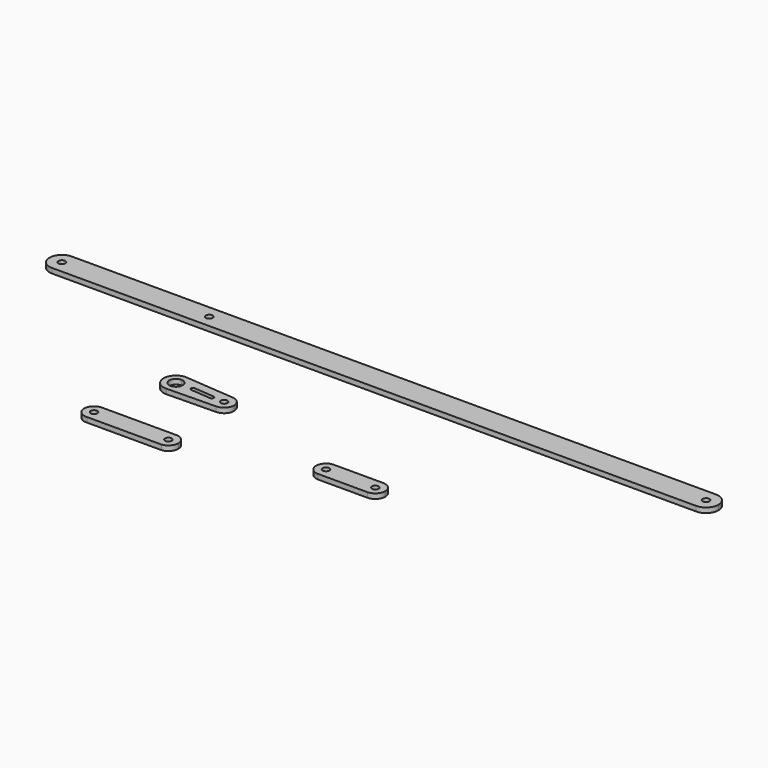
from build123d import *

# Parameters (mm, degrees)
F0_R     = 1.7399
F1_DEPTH = 2.54
F3_DEPTH = 2.54
F4_R     = 1.7145
F5_DEPTH = 2.54
F7_DEPTH = 2.54


# Not quite as in the source:
# - a feature names something its author has since deleted; it is built from what else it names


with BuildPart() as f1:
    # F0 (on Top) → F1 (new body)
    with BuildSketch(Plane.XY):
        with BuildLine():
            Line((-66.9744420796, 34.3977775435), (-71.5845430945, 34.3977775435))
            ThreePointArc((-71.5845430945, 34.3977775435), (-69.7246708578, 29.9076487653), (-65.2345420796, 28.0477765286))
            ThreePointArc((-65.2345420796, 28.0477765286), (-60.7444133014, 29.9076487653), (-58.8845410646, 34.3977775435))
            Line((-58.8845410646, 34.3977775435), (-63.4946420796, 34.3977775435))
            ThreePointArc((-63.4946420796, 34.3977775435), (-65.2345420796, 32.6578775435), (-66.9744420796, 34.3977775435))
        make_face()
        with BuildLine():
            ThreePointArc((-65.2345420796, 40.7477785584), (-69.7246708578, 38.8879063217), (-71.5845430945, 34.3977775435))
            Line((-71.5845430945, 34.3977775435), (-66.9744420796, 34.3977775435))
            ThreePointArc((-66.9744420796, 34.3977775435), (-65.2345420796, 36.1376775435), (-63.4946420796, 34.3977775435))
            Line((-63.4946420796, 34.3977775435), (-58.8845410646, 34.3977775435))
            ThreePointArc((-58.8845410646, 34.3977775435), (-60.7444133014, 38.8879063217), (-65.2345420796, 40.7477785584))
        make_face()
        with BuildLine():
            ThreePointArc((-140.7862693794, 28.0477775435), (-136.2961413189, 29.907649483), (-134.4362693794, 34.3977775435))
            ThreePointArc((-134.4362693794, 34.3977775435), (-136.2801574251, 38.8718646074), (-140.7409796332, 40.7476160327))
            ThreePointArc((-140.7409796332, 40.7476160327), (-147.1362290016, 34.4204225606), (-140.7862693794, 28.0477775435))
        make_face()
        with Locations((-140.7862693794, 34.3977775435)):
            Circle(F0_R, mode=Mode.SUBTRACT)
        with BuildLine():
            ThreePointArc((195.7637350565, 34.3977775435), (193.9038617876, 38.8879087708), (189.4137305353, 40.7477819794))
            ThreePointArc((189.4137305353, 40.7477819794), (184.9235993933, 38.8879087105), (183.0637261847, 34.3977775435))
            ThreePointArc((183.0637261847, 34.3977775435), (184.9235993933, 29.9076463765), (189.4137305353, 28.0477731076))
            ThreePointArc((189.4137305353, 28.0477731076), (193.9038617876, 29.9076463162), (195.7637350565, 34.3977775435))
        make_face()
        with BuildLine():
            ThreePointArc((191.1536306206, 34.3977775435), (189.4137306206, 32.6578775435), (187.6738306206, 34.3977775435))
            ThreePointArc((187.6738306206, 34.3977775435), (189.4137306206, 36.1376775435), (191.1536306206, 34.3977775435))
        make_face(mode=Mode.SUBTRACT)
        with BuildLine():
            Line((-71.5845430945, 34.3977775435), (-134.4362693794, 34.3977775435))
            ThreePointArc((-134.4362693794, 34.3977775435), (-136.2961413189, 29.907649483), (-140.7862693794, 28.0477775435))
            Line((-140.7862693794, 28.0477775435), (-65.2345420796, 28.0477765285))
            ThreePointArc((-65.2345420796, 28.0477765286), (-69.7246708578, 29.9076487653), (-71.5845430945, 34.3977775435))
        make_face()
        with BuildLine():
            ThreePointArc((-140.7409796332, 40.7476160327), (-136.2801574251, 38.8718646074), (-134.4362693794, 34.3977775435))
            Line((-134.4362693794, 34.3977775435), (-71.5845430945, 34.3977775435))
            ThreePointArc((-71.5845430945, 34.3977775435), (-69.7246708578, 38.8879063217), (-65.2345420796, 40.7477785584))
            Line((-65.2345420796, 40.7477785585), (-140.7409796332, 40.7476160327))
        make_face()
        with BuildLine():
            ThreePointArc((-58.8845410646, 34.3977775435), (-60.7444133014, 29.9076487653), (-65.2345420796, 28.0477765286))
            Line((-65.2345420796, 28.0477765285), (189.4137305353, 28.0477731076))
            ThreePointArc((189.4137305353, 28.0477731076), (184.9235993933, 29.9076463765), (183.0637261847, 34.3977775435))
            Line((183.0637261847, 34.3977775435), (-58.8845410646, 34.3977775435))
        make_face()
        with BuildLine():
            Line((189.4137305353, 40.7477819794), (-65.2345420796, 40.7477785585))
            ThreePointArc((-65.2345420796, 40.7477785584), (-60.7444133014, 38.8879063217), (-58.8845410646, 34.3977775435))
            Line((-58.8845410646, 34.3977775435), (183.0637261847, 34.3977775435))
            ThreePointArc((183.0637261847, 34.3977775435), (184.9235993933, 38.8879087105), (189.4137305353, 40.7477819794))
        make_face()
    extrude(amount=F1_DEPTH)


with BuildPart() as f3:
    # F2 (on Top) → F3 (new body)
    with BuildSketch(Plane.XY):
        with BuildLine():
            Line((-14.5032220102, -14.4440956048), (-38.7873029648, -12.4586465028))
            ThreePointArc((-38.7873029648, -12.4586465028), (-34.9776667278, -14.6150092623), (-33.4687510894, -18.7243160414))
            ThreePointArc((-33.4687510894, -18.7243160414), (-35.2214632817, -23.104663609), (-39.5120407945, -25.0669045346))
            Line((-39.5120407945, -25.0669045346), (-14.5032220102, -24.6210461602))
            ThreePointArc((-14.5032220102, -24.6210461602), (-19.5832220102, -19.5410461602), (-14.5032220102, -14.4610461602))
            Line((-14.5032220102, -14.4610461602), (-14.5032220102, -14.4440956048))
        make_face()
        with BuildLine():
            ThreePointArc((-20.7319625899, -18.5284234777), (-20.067623094, -18.8525118323), (-19.7987351869, -19.5410461602))
            ThreePointArc((-19.7987351869, -19.5410461602), (-20.0963146972, -20.2594666499), (-20.8147351869, -20.5570461602))
            ThreePointArc((-20.8147351869, -20.5570461602), (-20.8988618396, -20.5535572497), (-20.9824107159, -20.5431144797))
            Line((-20.9824107159, -20.5431144797), (-31.0041907261, -19.7104334206))
            ThreePointArc((-31.0041907261, -19.7104334206), (-32.1225060361, -18.6995983315), (-31.0041907261, -17.6887632424))
            Line((-31.0041907261, -17.6887632424), (-20.7319625899, -18.5284234777))
        make_face(mode=Mode.SUBTRACT)
        with BuildLine():
            Line((-39.8372522723, -15.2953659533), (-39.8187510894, -12.3743160414))
            ThreePointArc((-39.8187510894, -12.3743160414), (-46.1686237239, -18.6840975724), (-39.899186414, -25.0738065846))
            Line((-39.899186414, -25.0738065846), (-39.880685231, -22.1527566726))
            ThreePointArc((-39.880685231, -22.1527566726), (-43.247682312, -18.7025980681), (-39.8372522723, -15.2953659533))
        make_face()
        with BuildLine():
            Line((-38.7873029648, -12.4586465028), (-39.8187510894, -12.3743160414))
            Line((-39.8187510894, -12.3743160414), (-39.8372522723, -15.2953659533))
            ThreePointArc((-39.8372522723, -15.2953659533), (-37.4006319397, -16.2931145322), (-36.3897510894, -18.7243160414))
            ThreePointArc((-36.3897510894, -18.7243160414), (-37.4160787409, -21.1707842275), (-39.880685231, -22.1527566726))
            Line((-39.880685231, -22.1527566726), (-39.899186414, -25.0738065846))
            Line((-39.899186414, -25.0738065846), (-39.5120407945, -25.0669045346))
            ThreePointArc((-39.5120407945, -25.0669045346), (-35.2214632817, -23.104663609), (-33.4687510894, -18.7243160414))
            ThreePointArc((-33.4687510894, -18.7243160414), (-34.9776667278, -14.6150092623), (-38.7873029648, -12.4586465028))
        make_face()
        with BuildLine():
            ThreePointArc((-14.5032220102, -14.4610461602), (-19.5832220102, -19.5410461602), (-14.5032220102, -24.6210461602))
            Line((-14.5032220102, -24.6210461602), (-14.5032220102, -21.2555461602))
            ThreePointArc((-14.5032220102, -21.2555461602), (-16.2177220102, -19.5410461602), (-14.5032220102, -17.8265461602))
            Line((-14.5032220102, -17.8265461602), (-14.5032220102, -14.4610461602))
        make_face()
        with BuildLine():
            Line((-14.5032220102, -21.2555461602), (-14.5032220102, -24.6210461602))
            ThreePointArc((-14.5032220102, -24.6210461602), (-10.9111195618, -23.1331486087), (-9.4232220102, -19.5410461602))
            ThreePointArc((-9.4232220102, -19.5410461602), (-10.9111195618, -15.9489437118), (-14.5032220102, -14.4610461602))
            Line((-14.5032220102, -14.4610461602), (-14.5032220102, -17.8265461602))
            ThreePointArc((-14.5032220102, -17.8265461602), (-13.2908874339, -18.3287115839), (-12.7887220102, -19.5410461602))
            ThreePointArc((-12.7887220102, -19.5410461602), (-13.2908874339, -20.7533807366), (-14.5032220102, -21.2555461602))
        make_face()
    extrude(amount=F3_DEPTH)


with BuildPart() as f5:
    # F4 (on Top) → F5 (new body)
    with BuildSketch(Plane.XY):
        with BuildLine():
            ThreePointArc((53.9270043373, -44.8584560919), (57.5191067857, -43.3705585403), (59.0070043373, -39.7784560919))
            ThreePointArc((59.0070043373, -39.7784560919), (57.5191067857, -36.1863536435), (53.9270043373, -34.6984560919))
            ThreePointArc((53.9270043373, -34.6984560919), (48.8470043373, -39.7784560919), (53.9270043373, -44.8584560919))
        make_face()
        with Locations((53.9270043373, -39.7784560919)):
            Circle(F4_R, mode=Mode.SUBTRACT)
        with BuildLine():
            ThreePointArc((53.9270043373, -34.6984560919), (57.5191067857, -36.1863536435), (59.0070043373, -39.7784560919))
            Line((59.0070043373, -39.7784560919), (74.1077731681, -39.7784560919))
            ThreePointArc((74.1077731681, -39.7784560919), (75.5956707197, -36.1863536435), (79.1877731681, -34.6984560919))
            Line((79.1877731681, -34.6984560919), (53.9270043373, -34.6984560919))
        make_face()
        with BuildLine():
            Line((74.1077731681, -39.7784560919), (59.0070043373, -39.7784560919))
            ThreePointArc((59.0070043373, -39.7784560919), (57.5191067857, -43.3705585403), (53.9270043373, -44.8584560919))
            Line((53.9270043373, -44.8584560919), (79.1877731681, -44.8584560919))
            ThreePointArc((79.1877731681, -44.8584560919), (75.5956707197, -43.3705585403), (74.1077731681, -39.7784560919))
        make_face()
        with BuildLine():
            ThreePointArc((79.1877731681, -34.6984560919), (75.5956707197, -36.1863536435), (74.1077731681, -39.7784560919))
            ThreePointArc((74.1077731681, -39.7784560919), (75.5956707197, -43.3705585403), (79.1877731681, -44.8584560919))
            ThreePointArc((79.1877731681, -44.8584560919), (82.7798756165, -43.3705585403), (84.2677731681, -39.7784560919))
            ThreePointArc((84.2677731681, -39.7784560919), (82.7798756165, -36.1863536435), (79.1877731681, -34.6984560919))
        make_face()
        with BuildLine():
            ThreePointArc((80.9022731681, -39.7784560919), (79.1877731681, -41.4929560919), (77.4732731681, -39.7784560919))
            ThreePointArc((77.4732731681, -39.7784560919), (79.1877731681, -38.0639560919), (80.9022731681, -39.7784560919))
        make_face(mode=Mode.SUBTRACT)
    extrude(amount=F5_DEPTH)


with BuildPart() as f7:
    # F6 (on Top) → F7 (new body)
    with BuildSketch(Plane.XY):
        with BuildLine():
            ThreePointArc((-49.3108029973, -57.3654139877), (-48.2567317102, -57.9388698208), (-47.8368081551, -59.062961489))
            Line((-47.8368081551, -59.062961489), (-44.4713081551, -59.062961489))
            ThreePointArc((-44.4713081551, -59.062961489), (-45.9093825635, -55.5213830294), (-49.4094097241, -53.9849436832))
            Line((-49.4094097241, -53.9849436832), (-49.3108029973, -57.3654139877))
        make_face()
        with BuildLine():
            Line((-44.4713081551, -59.062961489), (-47.8368081551, -59.062961489))
            ThreePointArc((-47.8368081551, -59.062961489), (-48.2245068277, -60.1488291087), (-49.2122627922, -60.7436037745))
            Line((-49.2122627922, -60.7436037745), (-49.1136560654, -64.1240740789))
            ThreePointArc((-49.1136560654, -64.1240740789), (-45.8076687083, -62.4968461248), (-44.4713081551, -59.062961489))
        make_face()
        with BuildLine():
            ThreePointArc((-49.4094097241, -53.9849436832), (-45.9093825635, -55.5213830294), (-44.4713081551, -59.062961489))
            Line((-44.4713081551, -59.062961489), (-28.0248081551, -59.062961489))
            Line((-28.0248081551, -59.062961489), (-16.5313081551, -59.062961489))
            ThreePointArc((-16.5313081551, -59.062961489), (-15.0435043934, -55.4709528329), (-11.4515734366, -53.9829614959))
            Line((-11.4515734366, -53.9829614959), (-49.4094097241, -53.9849436832))
        make_face()
        with BuildLine():
            Line((-28.0248081551, -59.062961489), (-44.4713081551, -59.062961489))
            ThreePointArc((-44.4713081551, -59.062961489), (-45.8076687083, -62.4968461248), (-49.1136560654, -64.1240740789))
            Line((-49.1136560654, -64.1240740789), (-11.8889602447, -64.1240740789))
            ThreePointArc((-11.8889602447, -64.1240740789), (-15.1949476019, -62.4968461248), (-16.5313081551, -59.062961489))
            Line((-16.5313081551, -59.062961489), (-28.0248081551, -59.062961489))
        make_face()
        with BuildLine():
            ThreePointArc((-49.2122627922, -60.7436037745), (-51.2650792192, -59.1129513838), (-49.3108029973, -57.3654139877))
            Line((-49.3108029973, -57.3654139877), (-49.4094097241, -53.9849436832))
            ThreePointArc((-49.4094097241, -53.9849436832), (-54.6291483452, -59.2110796959), (-49.1136560654, -64.1240740789))
            Line((-49.1136560654, -64.1240740789), (-49.2122627922, -60.7436037745))
        make_face()
        with BuildLine():
            ThreePointArc((-11.4515734366, -53.9829614959), (-15.0435043934, -55.4709528329), (-16.5313081551, -59.062961489))
            Line((-16.5313081551, -59.062961489), (-13.1658081551, -59.062961489))
            ThreePointArc((-13.1658081551, -59.062961489), (-12.6111226715, -57.8002895056), (-11.3059766736, -57.3546321851))
            Line((-11.3059766736, -57.3546321851), (-11.4515734366, -53.9829614959))
        make_face()
        with BuildLine():
            Line((-13.1658081551, -59.062961489), (-16.5313081551, -59.062961489))
            ThreePointArc((-16.5313081551, -59.062961489), (-15.1949476019, -62.4968461248), (-11.8889602447, -64.1240740789))
            Line((-11.8889602447, -64.1240740789), (-11.0136560654, -64.1240740789))
            Line((-11.0136560654, -64.1240740789), (-11.1592528283, -60.7524033897))
            ThreePointArc((-11.1592528283, -60.7524033897), (-12.5555684034, -60.3744947725), (-13.1658081551, -59.062961489))
        make_face()
        with BuildLine():
            ThreePointArc((-6.3713081551, -59.062961489), (-7.859299499, -55.4707652506), (-11.4515734366, -53.9829614959))
            Line((-11.4515734366, -53.9829614959), (-11.3059766736, -57.3546321851))
            ThreePointArc((-11.3059766736, -57.3546321851), (-10.1886361717, -57.9031469725), (-9.7368081551, -59.062961489))
            ThreePointArc((-9.7368081551, -59.062961489), (-10.1397748715, -60.1672217374), (-11.1592528283, -60.7524033897))
            Line((-11.1592528283, -60.7524033897), (-11.0136560654, -64.1240740789))
            ThreePointArc((-11.0136560654, -64.1240740789), (-7.7076687083, -62.4968461248), (-6.3713081551, -59.062961489))
        make_face()
    extrude(amount=F7_DEPTH)


solid = Compound([f1.part, f3.part, f5.part, f7.part])
